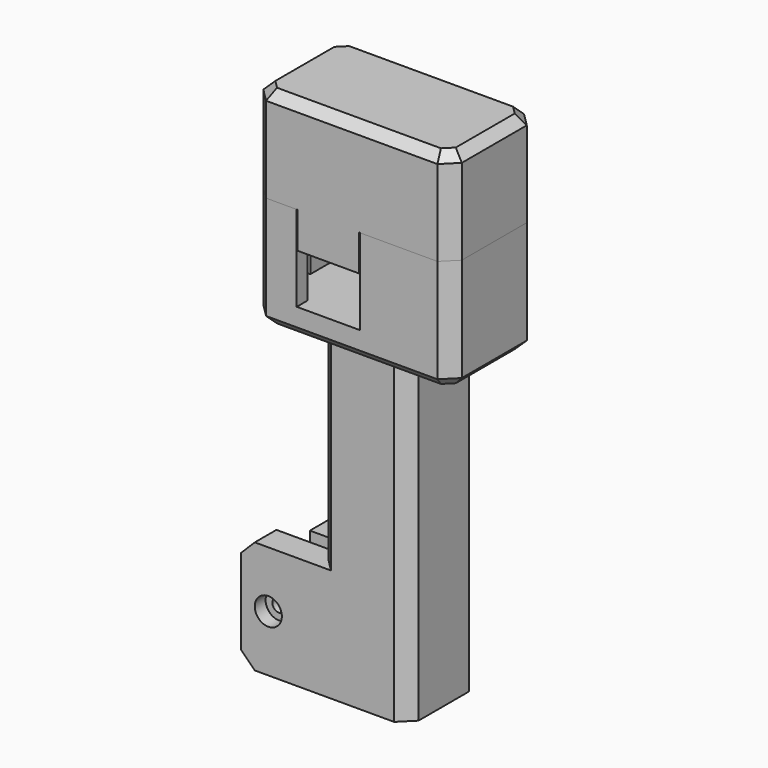
from build123d import *

# Parameters (mm, degrees)
F1_DEPTH   = 12.5
F2_R       = 1.5
F3_DEPTH   = 6
F4_R       = 3
F5_DEPTH   = 3
F7_DEPTH   = 10.6
F8_W       = 20
F8_H       = 20
F9_DEPTH   = 45
F10_R      = 1.55
F11_DEPTH  = 20
F12_SIZE   = 3
F13_W      = 44
F13_H      = 24
F14_DEPTH  = 6
F16_DEPTH  = 19
F18_DEPTH  = 3
F19_SIZE   = 3
F21_DEPTH  = 19
F23_DEPTH  = 2
F24_W      = 13.6
F24_H      = 8
F25_DEPTH  = 3
F27_DEPTH  = 3
F28_SIZE   = 2
F28_2_SIZE = 2
F29_R      = 1.7
F30_DEPTH  = 6
F31_R      = 3.2
F32_DEPTH  = 3
F33_SIZE   = 3


with BuildPart() as f1:
    # F0 (on Top) → F1 (new body, symmetric)
    with BuildSketch(Plane.XY):
        Polygon((30.9, 14), (1.7, 14), (1.7, 3.4), (10.9, 3.4), (10.9, 0), (-6, 0), (-6, -6), (30.9, -6), align=None)
    extrude(amount=F1_DEPTH, both=True)

    # F2 (on face) → F3 (cut, through all)
    with BuildSketch(Plane.XZ.offset(6)):
        Circle(F2_R)
    extrude(amount=-F3_DEPTH, mode=Mode.SUBTRACT)

    # F4 (on face) → F5 (cut)
    with BuildSketch(Plane.XZ.offset(6)):
        Circle(F4_R)
    extrude(amount=-F5_DEPTH, mode=Mode.SUBTRACT)

    # F6 (on face) → F7 (cut, through all)
    with BuildSketch(Plane.XZ.offset(-3.4)):
        Polygon((5, -2.8867513459), (5, 2.8867513459), (0, 5.7735026919), (-5, 2.8867513459), (-5, -2.8867513459), (0, -5.7735026919), align=None)
    extrude(amount=-F7_DEPTH, mode=Mode.SUBTRACT)

    # F8 (on face) → F9 (join)
    with BuildSketch(Plane.XY.offset(12.5)):
        with Locations((20.9, 4)):
            Rectangle(F8_W, F8_H)
    extrude(amount=F9_DEPTH)

    # F10 (on face) → F11 (cut)
    with BuildSketch(Plane.XY.offset(57.5)):
        with Locations((20.9, 4)):
            Circle(F10_R)
    extrude(amount=-F11_DEPTH, mode=Mode.SUBTRACT)

    # F12
    f12_edges = [f1.edges().sort_by_distance(p)[0] for p in [
        (10.9, 14, 35),
        (10.9, -6, 35),
        (30.9, -6, 22.5),
        (30.9, 14, 22.5),
    ]]
    chamfer(f12_edges, length=F12_SIZE)

    # F33
    f33_edges = [f1.edges().sort_by_distance(p)[0] for p in [
        (-6, -3, 12.5),
        (-6, -3, -12.5),
    ]]
    chamfer(f33_edges, length=F33_SIZE)


with BuildPart() as f14:
    # F13 (on face) → F14 (new body)
    with BuildSketch(Plane.XY.offset(57.5)):
        with Locations((20.9, 3)):
            Rectangle(F13_W, F13_H)
    extrude(amount=F14_DEPTH)

    # F15 (on face) → F16 (join)
    with BuildSketch(Plane.XY.offset(63.5)):
        Polygon((11.9, 12), (11.9, 15), (-1.1, 15), (-1.1, -9), (8.7, -9), (8.7, -6), (2.9, -6), (2.9, -0.2), (1.7, -0.2), (1.7, 2), (2.9, 2), (2.9, 12), align=None)
        Polygon((42.9, 15), (29.9, 15), (29.9, 12), (38.9, 12), (38.9, 2), (40.1, 2), (40.1, -0.2), (38.9, -0.2), (38.9, -6), (22.7, -6), (22.7, -9), (42.9, -9), align=None)
    extrude(amount=F16_DEPTH)

    # F17 (on face) → F18 (join, through all)
    with BuildSketch(Plane(origin=(0, 15, 0), x_dir=(-1, 0, 0), z_dir=(0, 1, 0))):
        with BuildLine():
            ThreePointArc((-11.9, 82.5), (-20.9, 73.5), (-29.9, 82.5))
            Line((-29.9, 82.5), (-29.9, 63.5))
            Line((-29.9, 63.5), (-11.9, 63.5))
            Line((-11.9, 63.5), (-11.9, 82.5))
        make_face()
    extrude(amount=-F18_DEPTH)

    # F19
    f19_edges = [f14.edges().sort_by_distance(p)[0] for p in [
        (42.9, 15, 70),
        (-1.1, 15, 70),
        (-1.1, -9, 70),
        (42.9, -9, 70),
    ]]
    chamfer(f19_edges, length=F19_SIZE)

    # F28
    f28_edges = [f14.edges().sort_by_distance(p)[0] for p in [
        (20.9, 15, 57.5),
        (41.4, 13.5, 57.5),
        (0.4, 13.5, 57.5),
        (42.9, 3, 57.5),
        (-1.1, 3, 57.5),
        (41.4, -7.5, 57.5),
        (0.4, -7.5, 57.5),
        (20.9, -9, 57.5),
    ]]
    chamfer(f28_edges, length=F28_SIZE)

    # F29 (on face) → F30 (cut, through all)
    with BuildSketch(Plane.XY.offset(63.5)):
        with Locations((20.9, 4)):
            Circle(F29_R)
    extrude(amount=-F30_DEPTH, mode=Mode.SUBTRACT)

    # F31 (on face) → F32 (cut)
    with BuildSketch(Plane.XY.offset(63.5)):
        with Locations((20.9, 4)):
            Circle(F31_R)
    extrude(amount=-F32_DEPTH, mode=Mode.SUBTRACT)


with BuildPart() as f21:
    # F20 (on face) → F21 (new body)
    with BuildSketch(Plane.XY.offset(82.5)):
        Polygon((11.9, 15), (1.9, 15), (-1.1, 12), (-1.1, -6), (1.9, -9), (8.7, -9), (8.7, -6), (2.9, -6), (2.9, -0.2), (1.7, -0.2), (1.7, 2), (2.9, 2), (2.9, 12), (11.9, 12), align=None)
    extrude(amount=F21_DEPTH)



with BuildPart() as f21b:
    # F20 (on face) → F21, piece 2 (new body)
    with BuildSketch(Plane.XY.offset(82.5)):
        Polygon((42.9, 12), (39.9, 15), (29.9, 15), (29.9, 12), (38.9, 12), (38.9, 2), (40.1, 2), (40.1, -0.2), (38.9, -0.2), (38.9, -6), (22.7, -6), (22.7, -9), (39.9, -9), (42.9, -6), align=None)
    extrude(amount=F21_DEPTH)


with BuildPart() as f21_1:
    add(f21.part)

    add(f21b.part)  # F23 merges F21b
    # F22 (on face) → F23 (join)
    with BuildSketch(Plane.XY.offset(101.5)):
        Polygon((39.9, 15), (1.9, 15), (-1.1, 12), (-1.1, -6), (1.9, -9), (39.9, -9), (42.9, -6), (42.9, 12), align=None)
    extrude(amount=F23_DEPTH)

    # F24 (on face) → F25 (join, through all)
    with BuildSketch(Plane.XZ.offset(9)):
        Polygon((22.7, 101.5), (8.7, 101.5), (8.7, 82.5), (8.9, 82.5), (22.5, 82.5), (22.7, 82.5), align=None)
        with Locations((15.7, 78.5)):
            Rectangle(F24_W, F24_H)
    extrude(amount=-F25_DEPTH)

    # F26 (on face) → F27 (join, through all)
    with BuildSketch(Plane(origin=(0, 15, 0), x_dir=(-1, 0, 0), z_dir=(0, 1, 0))):
        with BuildLine():
            ThreePointArc((-29.9, 82.5), (-20.9, 91.5), (-11.9, 82.5))
            Line((-11.9, 82.5), (-11.9, 101.5))
            Line((-11.9, 101.5), (-29.9, 101.5))
            Line((-29.9, 101.5), (-29.9, 82.5))
        make_face()
    extrude(amount=-F27_DEPTH)

    # F28#2
    f28_2_edges = [f21_1.edges().sort_by_distance(p)[0] for p in [
        (20.9, 15, 103.5),
        (0.4, 13.5, 103.5),
        (-1.1, 3, 103.5),
        (0.4, -7.5, 103.5),
        (20.9, -9, 103.5),
        (41.4, -7.5, 103.5),
        (42.9, 3, 103.5),
        (41.4, 13.5, 103.5),
    ]]
    chamfer(f28_2_edges, length=F28_2_SIZE)


solid = Compound([f1.part, f14.part, f21_1.part])
